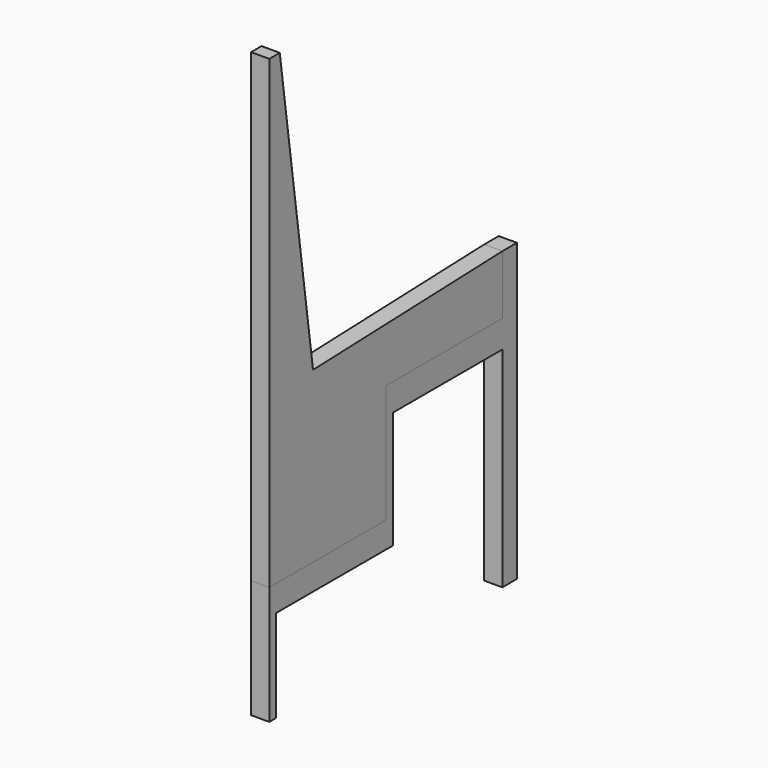
from build123d import *

# Parameters (mm, degrees)
F1_DEPTH = 25.4
F2_DEPTH = 25.4


# Not quite as in the source:
# - a feature names something its author has since deleted; it is built from what else it names


with BuildPart() as f1:
    # F0 (on Right) → F1 (new body)
    with BuildSketch(Plane.YZ):
        Polygon((0, 203.2), (0, 165.1), (203.2, 165.1), (203.2, 330.2), (406.4, 330.2), (406.4, 412.75), (76.288649265, 401.2222576144), (74.6685307278, 412.75), (0, 412.75), (0, 330.2), align=None)
        Polygon((0, 814.1079739114), (0, 412.75), (74.6685307278, 412.75), (18.2613460599, 814.1079739114), align=None)
    extrude(amount=F1_DEPTH)


with BuildPart() as f2:
    # F0 (on Right) → F2 (new body)
    with BuildSketch(Plane.YZ):
        Polygon((406.4, 412.75), (406.4, 330.2), (406.4, 292.1), (406.4, 0), (431.8, 0), (431.8, 412.75), align=None)
        Polygon((0, 165.1), (0, 0), (11.8412161246, 0), (11.8412161246, 128.8679540157), (203.2, 128.8679540157), (215.9764766693, 128.8679540157), (215.9764766693, 292.1), (406.4, 292.1), (406.4, 330.2), (203.2, 330.2), (203.2, 165.1), align=None)
    extrude(amount=F2_DEPTH)


solid = Compound([f1.part, f2.part])
